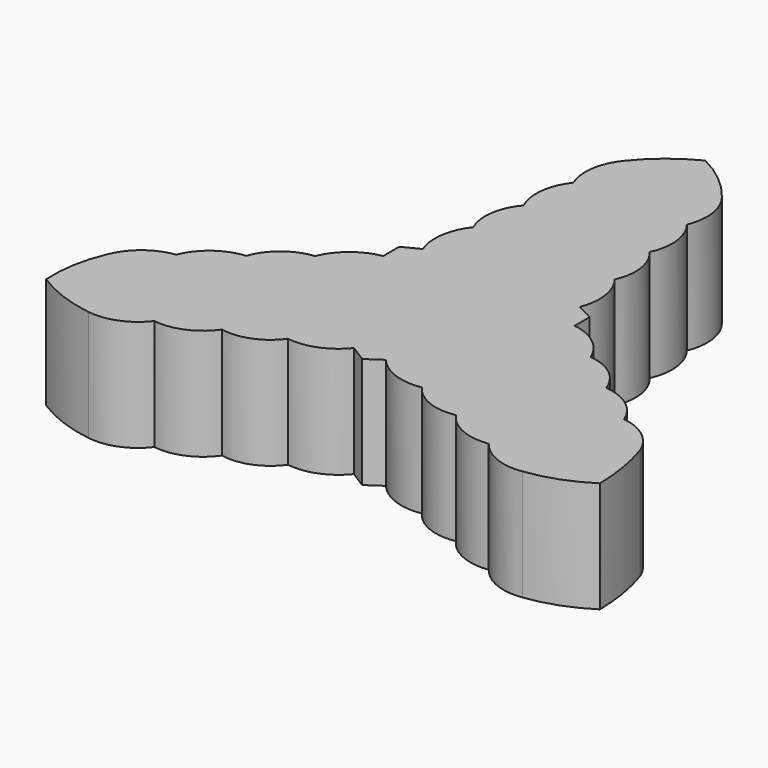
from build123d import *

# Parameters (mm, degrees)
F1_DEPTH = 14.2875


# Not quite as in the source:
# - a length typed as a fraction of an inch, garbled in the dataset ("3 / 203.2 mm" for 3/8 in), is restored


with BuildPart() as f1:
    # F0 (on Top) → F1 (new body)
    with BuildSketch(Plane.XY):
        with BuildLine():
            ThreePointArc((-0.0584694644, 41.0366132855), (-3.5379130554, 38.7889545067), (-6.4473585226, 35.840459168))
            ThreePointArc((-6.4473585226, 35.840459168), (-7.8691085687, 32.5448223466), (-7.4162920937, 28.9842672646))
            ThreePointArc((-7.4162920937, 28.9842672646), (-8.8119305122, 25.5953281623), (-8.2258973271, 21.977417171))
            ThreePointArc((-8.2258973271, 21.977417171), (-9.7181261566, 18.698842434), (-9.2097157612, 15.1327075437))
            ThreePointArc((-9.2097157612, 15.1327075437), (-10.6205392688, 11.8246856933), (-10.2093555033, 8.2519613206))
            Line((-10.2093555033, 8.2519613206), (-12.369341217, 7.1464567445))
            Line((-12.369341217, 7.1464567445), (-12.369341217, 4.6386048198))
            Line((-12.369341217, 4.6386048198), (-12.369341217, 4.5682978211))
            ThreePointArc((-12.369341217, 4.5682978211), (-15.5930977879, 3.1185654947), (-17.7027139134, 0.2823972963))
            ThreePointArc((-17.7027139134, 0.2823972963), (-21.0452825194, -1.0603738309), (-23.1384971151, -3.9919692741))
            ThreePointArc((-23.1384971151, -3.9919692741), (-26.5647165348, -5.2934051439), (-28.80180468, -8.19653302))
            ThreePointArc((-28.80180468, -8.19653302), (-32.1117440701, -9.5846599904), (-34.254974256, -12.4637500588))
            ThreePointArc((-34.254974256, -12.4637500588), (-35.4454588739, -16.4293701566), (-35.6585793197, -20.564340055))
            ThreePointArc((-35.6585793197, -20.564340055), (-31.9389059128, -22.4150036937), (-27.9142765499, -23.4461606411))
            ThreePointArc((-27.9142765499, -23.4461606411), (-24.3492963179, -23.0296138883), (-21.4921734029, -20.8571857766))
            ThreePointArc((-21.4921734029, -20.8571857766), (-17.8594468391, -20.3713745504), (-15.0192606046, -18.054899429))
            ThreePointArc((-15.0192606046, -18.054899429), (-11.4338171794, -17.7079201351), (-8.5996589687, -15.484556372))
            ThreePointArc((-8.5996589687, -15.484556372), (-5.0294162563, -15.0523544446), (-2.1409380715, -12.9098966718))
            Line((-2.1409380715, -12.9098966718), (0, -14.2561570176))
            Line((0, -14.2561570176), (1.9696742658, -12.9098966718))
            ThreePointArc((1.9696742658, -12.9098966718), (4.9392756736, -15.0084468105), (8.560301624, -15.3410370587))
            ThreePointArc((8.560301624, -15.3410370587), (11.3944598347, -17.5644008218), (14.9799032599, -17.9113801157))
            ThreePointArc((14.9799032599, -17.9113801157), (17.8200894944, -20.2278552371), (21.4528160582, -20.7136664634))
            ThreePointArc((21.4528160582, -20.7136664634), (24.3099389732, -22.886094575), (27.8749192052, -23.3026413279))
            ThreePointArc((27.8749192052, -23.3026413279), (31.8832272801, -22.3269581873), (35.5659238994, -20.4678624868))
            ThreePointArc((35.5659238994, -20.4678624868), (35.2059818343, -16.3418066269), (34.2156169113, -12.3202307456))
            ThreePointArc((34.2156169113, -12.3202307456), (32.0723867254, -9.4411406771), (28.7624473353, -8.0530137067))
            ThreePointArc((28.7624473353, -8.0530137067), (26.5253591901, -5.1498858306), (23.0991397704, -3.8484499608))
            ThreePointArc((23.0991397704, -3.8484499608), (21.0059251747, -0.9168545176), (17.6633565687, 0.4259166096))
            ThreePointArc((17.6633565687, 0.4259166096), (15.4847616458, 3.3168082822), (12.1560195839, 4.739132713))
            Line((12.1560195839, 4.739132713), (12.1560195839, 7.1464567445))
            Line((12.1560195839, 7.1464567445), (9.9960338703, 8.2519613206))
            ThreePointArc((9.9960338703, 8.2519613206), (10.4072176357, 11.8246856933), (8.9963941282, 15.1327075437))
            ThreePointArc((8.9963941282, 15.1327075437), (9.5048045235, 18.698842434), (8.012575694, 21.977417171))
            ThreePointArc((8.012575694, 21.977417171), (8.5986088792, 25.5953281623), (7.2029704606, 28.9842672646))
            ThreePointArc((7.2029704606, 28.9842672646), (7.6557869357, 32.5448223466), (6.2340368895, 35.840459168))
            ThreePointArc((6.2340368895, 35.840459168), (3.3823120514, 38.7952079886), (-0.0584694644, 41.0366132855))
        make_face()
    extrude(amount=F1_DEPTH)


solid = f1.part
